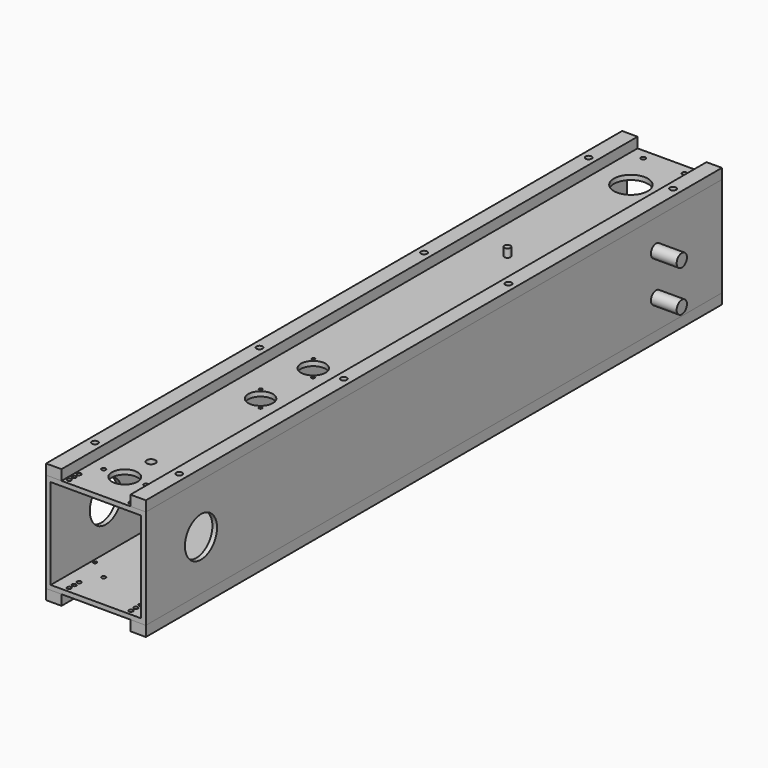
from build123d import *

# Parameters (mm, degrees)
F0_W           = 97
F0_H           = 97
F0_W_2         = 88
F0_H_2         = 88
F1_DEPTH       = 700
F2_W           = 15
F2_H           = 700
F3_DEPTH       = 10
F4_W           = 15
F4_H           = 700
F5_DEPTH       = 10
F6_R           = 12.5
F6_R_2         = 12
F6_R_3         = 1.5
F7_DEPTH       = 25
F6_R_4         = 4.25
F6_R_5         = 2
F8_DEPTH       = 150
F9_R           = 12
F9_R_2         = 1.5
F10_DEPTH      = 25
F11_R          = 19.5
F11_R_2        = 6.26
F12_DEPTH      = 150
F13_DEPTH      = 150
F6_R_6         = 2.25
F14_DEPTH      = 150
F6_R_7         = 16.5
F15_DEPTH      = 50
F16_DEPTH      = 122
F16_DEPTH_BACK = 25
F17_DEPTH      = 122
F17_DEPTH_BACK = 25
F18_R          = 1.75
F19_DEPTH      = 150
F18_R_2        = 3
F20_DEPTH      = 5
F21_R          = 3
F21_R_2        = 1.75
F22_DEPTH      = 5
F6_R_8         = 3
F23_DEPTH      = 120
F24_DEPTH      = 8
F24_DEPTH_BACK = 105
F25_DEPTH      = 150


with BuildPart() as f1:
    # F0 (on Front) → F1 (new body)
    with BuildSketch(Plane.XZ):
        with Locations((48.5, 48.5)):
            Rectangle(F0_W, F0_H)
        with Locations((48.5, 48.5)):
            Rectangle(F0_W_2, F0_H_2, mode=Mode.SUBTRACT)
    extrude(amount=F1_DEPTH)

    # F6 (on face) → F7 (cut)
    with BuildSketch(Plane.XY.offset(97)):
        with Locations((48.5, -665)):
            Circle(F6_R)
        with Locations((48.5, -500)):
            Circle(F6_R_2)
        with Locations((48.5, -436)):
            Circle(F6_R_2)
        with Locations((58, -448)):
            Circle(F6_R_3)
        with Locations((39, -424)):
            Circle(F6_R_3)
        with Locations((39, -488)):
            Circle(F6_R_3)
        with Locations((58, -512)):
            Circle(F6_R_3)
    extrude(amount=-F7_DEPTH, mode=Mode.SUBTRACT)

    # F6 (on face) → F8 (cut)
    with BuildSketch(Plane.XY.offset(97)):
        with Locations((48.5, -633)):
            Circle(F6_R_4)
        with Locations((69, -665)):
            Circle(F6_R_5)
        with Locations((28, -665)):
            Circle(F6_R_5)
    extrude(amount=-F8_DEPTH, mode=Mode.SUBTRACT)

    # F9 (on face) → F10 (cut)
    with BuildSketch(Plane(origin=(0, 0, 0), x_dir=(1, 0, 0), z_dir=(0, 0, -1))):
        with Locations((48.5, 468)):
            Circle(F9_R)
        with Locations((39, 480)):
            Circle(F9_R_2)
        with Locations((58, 456)):
            Circle(F9_R_2)
        with Locations((48.5, 404)):
            Circle(F9_R)
        with Locations((58, 392)):
            Circle(F9_R_2)
        with Locations((39, 416)):
            Circle(F9_R_2)
    extrude(amount=-F10_DEPTH, mode=Mode.SUBTRACT)

    # F11 (on face) → F12 (cut)
    with BuildSketch(Plane.YZ.offset(97)):
        with Locations((-633, 48.5)):
            Circle(F11_R)
        with Locations((-80, 68.5)):
            Circle(F11_R_2)
        with Locations((-80, 28.5)):
            Circle(F11_R_2)
    extrude(amount=-F12_DEPTH, mode=Mode.SUBTRACT)

    # F6 (on face) → F13 (cut)
    with BuildSketch(Plane.XY.offset(97)):
        with BuildLine():
            ThreePointArc((16.5, -683), (18.5, -685), (20.5, -683))
            ThreePointArc((20.5, -683), (18.5, -681), (16.5, -683))
        make_face()
        with BuildLine():
            ThreePointArc((76.5, -683), (78.5, -685), (80.5, -683))
            ThreePointArc((80.5, -683), (78.5, -681), (76.5, -683))
        make_face()
    extrude(amount=-F13_DEPTH, mode=Mode.SUBTRACT)

    # F6 (on face) → F14 (cut)
    with BuildSketch(Plane.XY.offset(97)):
        with Locations((28.5, -10)):
            Circle(F6_R_6)
        with Locations((68.5, -10)):
            Circle(F6_R_6)
    extrude(amount=-F14_DEPTH, mode=Mode.SUBTRACT)

    # F6 (on face) → F15 (cut)
    with BuildSketch(Plane.XY.offset(97)):
        with Locations((48.5, -50)):
            Circle(F6_R_7)
    extrude(amount=-F15_DEPTH, mode=Mode.SUBTRACT)


with BuildPart() as f3:
    # F2 (on face) → F3 (new body)
    with BuildSketch(Plane.XY.offset(97)):
        with Locations((7.5, -350)):
            Rectangle(F2_W, F2_H)
    extrude(amount=F3_DEPTH)


with BuildPart() as f3b:
    # F2 (on face) → F3, piece 2 (new body)
    with BuildSketch(Plane.XY.offset(97)):
        with Locations((89.5, -350)):
            Rectangle(F2_W, F2_H)
    extrude(amount=F3_DEPTH)


with BuildPart() as f5:
    # F4 (on face) → F5 (new body)
    with BuildSketch(Plane(origin=(0, 0, 0), x_dir=(1, 0, 0), z_dir=(0, 0, -1))):
        with Locations((7.5, 350)):
            Rectangle(F4_W, F4_H)
    extrude(amount=F5_DEPTH)


with BuildPart() as f5b:
    # F4 (on face) → F5, piece 2 (new body)
    with BuildSketch(Plane(origin=(0, 0, 0), x_dir=(1, 0, 0), z_dir=(0, 0, -1))):
        with Locations((89.5, 350)):
            Rectangle(F4_W, F4_H)
    extrude(amount=F5_DEPTH)


with BuildPart() as f16:
    # F11 (on face) → F16 (new body, two sides)
    with BuildSketch(Plane.YZ.offset(97)) as f16_sk:
        with Locations((-80, 68.5)):
            Circle(F11_R_2)
    extrude(amount=-F16_DEPTH)
    extrude(f16_sk.sketch, amount=F16_DEPTH_BACK)


with BuildPart() as f17:
    # F11 (on face) → F17 (new body, two sides)
    with BuildSketch(Plane.YZ.offset(97)) as f17_sk:
        with Locations((-80, 28.5)):
            Circle(F11_R_2)
    extrude(amount=-F17_DEPTH)
    extrude(f17_sk.sketch, amount=F17_DEPTH_BACK)


with BuildPart() as f19_tool:
    # F18 (on face) → F19 (new body)
    with BuildSketch(Plane.XY.offset(107)):
        with Locations((7.5, -650)):
            Circle(F18_R)
        with Locations((7.5, -450)):
            Circle(F18_R)
        with Locations((7.5, -250)):
            Circle(F18_R)
        with Locations((7.5, -50)):
            Circle(F18_R)
        with Locations((89.5, -50)):
            Circle(F18_R)
        with Locations((89.5, -250)):
            Circle(F18_R)
        with Locations((89.5, -450)):
            Circle(F18_R)
        with Locations((89.5, -650)):
            Circle(F18_R)
    extrude(amount=-F19_DEPTH)


with BuildPart() as f1_1:
    add(f1.part)

    # F19: cut by f19_tool
    add(f19_tool.part, mode=Mode.SUBTRACT)

    # F6 (on face) → F23 (cut)
    with BuildSketch(Plane.XY.offset(97)):
        with Locations((48.5, -200)):
            Circle(F6_R_8)
    extrude(amount=-F23_DEPTH, mode=Mode.SUBTRACT)

    # F6 (on face) → F24 (join, two sides)
    with BuildSketch(Plane.XY.offset(97)) as f24_sk:
        with Locations((48.5, -200)):
            Circle(F6_R_8)
    extrude(amount=F24_DEPTH)
    extrude(f24_sk.sketch, amount=-F24_DEPTH_BACK)

    # F6 (on face) → F25 (cut)
    with BuildSketch(Plane.XY.offset(97)):
        with BuildLine():
            ThreePointArc((20.5, -695), (18.5, -693), (16.5, -695))
            ThreePointArc((16.5, -695), (18.5, -697), (20.5, -695))
        make_face()
        with BuildLine():
            ThreePointArc((80.5, -695), (78.5, -693), (76.5, -695))
            ThreePointArc((76.5, -695), (78.5, -697), (80.5, -695))
        make_face()
        with Locations((18.5, -689)):
            Circle(F6_R_5)
        with Locations((78.5, -689)):
            Circle(F6_R_5)
    extrude(amount=-F25_DEPTH, mode=Mode.SUBTRACT)


with BuildPart() as f3_1:
    add(f3.part)

    # F19: cut by f19_tool
    add(f19_tool.part, mode=Mode.SUBTRACT)


with BuildPart() as f3b_1:
    add(f3b.part)

    # F19: cut by f19_tool
    add(f19_tool.part, mode=Mode.SUBTRACT)


with BuildPart() as f5_1:
    add(f5.part)

    # F19: cut by f19_tool
    add(f19_tool.part, mode=Mode.SUBTRACT)


with BuildPart() as f5b_1:
    add(f5b.part)

    # F19: cut by f19_tool
    add(f19_tool.part, mode=Mode.SUBTRACT)


with BuildPart() as f20_tool:
    # F18 (on face) → F20 (new body)
    with BuildSketch(Plane.XY.offset(107)):
        with Locations((7.5, -650)):
            Circle(F18_R_2)
        with Locations((7.5, -650)):
            Circle(F18_R, mode=Mode.SUBTRACT)
        with Locations((89.5, -650)):
            Circle(F18_R_2)
        with Locations((89.5, -650)):
            Circle(F18_R, mode=Mode.SUBTRACT)
        with Locations((7.5, -450)):
            Circle(F18_R_2)
        with Locations((7.5, -450)):
            Circle(F18_R, mode=Mode.SUBTRACT)
        with Locations((89.5, -450)):
            Circle(F18_R_2)
        with Locations((89.5, -450)):
            Circle(F18_R, mode=Mode.SUBTRACT)
        with Locations((7.5, -250)):
            Circle(F18_R_2)
        with Locations((7.5, -250)):
            Circle(F18_R, mode=Mode.SUBTRACT)
        with Locations((89.5, -250)):
            Circle(F18_R_2)
        with Locations((89.5, -250)):
            Circle(F18_R, mode=Mode.SUBTRACT)
        with Locations((7.5, -50)):
            Circle(F18_R_2)
        with Locations((7.5, -50)):
            Circle(F18_R, mode=Mode.SUBTRACT)
        with Locations((89.5, -50)):
            Circle(F18_R_2)
        with Locations((89.5, -50)):
            Circle(F18_R, mode=Mode.SUBTRACT)
    extrude(amount=-F20_DEPTH)


with BuildPart() as f3_2:
    add(f3_1.part)

    # F20: cut by f20_tool
    add(f20_tool.part, mode=Mode.SUBTRACT)


with BuildPart() as f3b_2:
    add(f3b_1.part)

    # F20: cut by f20_tool
    add(f20_tool.part, mode=Mode.SUBTRACT)


with BuildPart() as f22_tool:
    # F21 (on face) → F22 (new body)
    with BuildSketch(Plane(origin=(0, 0, -10), x_dir=(1, 0, 0), z_dir=(0, 0, -1))):
        with Locations((89.5, 50)):
            Circle(F21_R)
        with Locations((89.5, 50)):
            Circle(F21_R_2, mode=Mode.SUBTRACT)
        with Locations((7.5, 50)):
            Circle(F21_R)
        with Locations((89.5, 250)):
            Circle(F21_R)
        with Locations((89.5, 250)):
            Circle(F21_R_2, mode=Mode.SUBTRACT)
        with Locations((7.5, 250)):
            Circle(F21_R)
        with Locations((7.5, 450)):
            Circle(F21_R)
        with Locations((89.5, 450)):
            Circle(F21_R)
        with Locations((89.5, 450)):
            Circle(F21_R_2, mode=Mode.SUBTRACT)
        with Locations((7.5, 650)):
            Circle(F21_R)
        with Locations((89.5, 650)):
            Circle(F21_R)
        with Locations((89.5, 650)):
            Circle(F21_R_2, mode=Mode.SUBTRACT)
    extrude(amount=-F22_DEPTH)


with BuildPart() as f5_2:
    add(f5_1.part)

    # F22: cut by f22_tool
    add(f22_tool.part, mode=Mode.SUBTRACT)


with BuildPart() as f5b_2:
    add(f5b_1.part)

    # F22: cut by f22_tool
    add(f22_tool.part, mode=Mode.SUBTRACT)


solid = Compound([f16.part, f17.part, f1_1.part, f3_2.part, f3b_2.part, f5_2.part, f5b_2.part])
